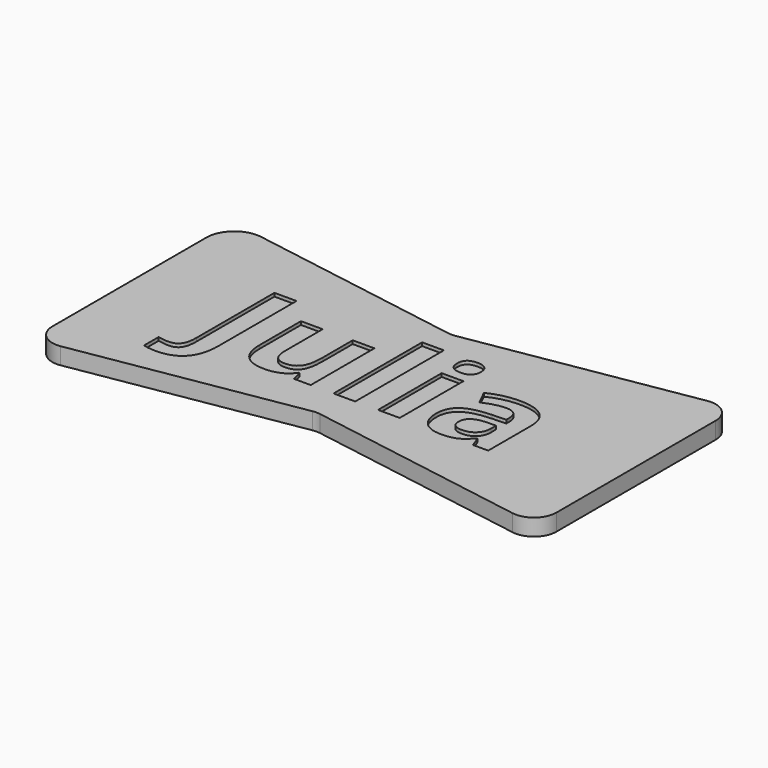
from build123d import *

# Parameters (mm, degrees)
F1_DEPTH     = 3
F2_TEXT_SIZE = 26.0301089535
F3_DEPTH     = 0.6


# Not quite as in the source:
# - Text() gives the source's letters only with a copy of the font that has no kerning and outlines rounded to 1/6400 em; it was checked with that copy


with BuildPart() as f1:
    # F0 (on Top) → F1 (new body)
    with BuildSketch(Plane.XY):
        with BuildLine():
            ThreePointArc((-40.8889098256, 19.2117940781), (-44.9427792428, 18.0949243713), (-46.7109047621, 14.2798244589))
            Line((-46.7109047621, 14.2798244589), (-46.7109047621, -20.0960317456))
            ThreePointArc((-46.7109047621, -20.0960317456), (-45.2964043467, -23.1481116755), (-42.0533088129, -24.041607441))
            Line((-42.0533088129, -24.041607441), (-2.3685007114, -17.4274727574))
            ThreePointArc((-2.3685007114, -17.4274727574), (-1.7109047621, -17.3730484527), (-1.0533088129, -17.4274727574))
            Line((-1.0533088129, -17.4274727574), (38.6314992886, -24.041607441))
            ThreePointArc((38.6314992886, -24.041607441), (41.8745948224, -23.1481116755), (43.2890952379, -20.0960317456))
            Line((43.2890952379, -20.0960317456), (43.2890952379, 15.4602848806))
            ThreePointArc((43.2890952379, 15.4602848806), (41.8745948224, 18.5123648105), (38.6314992886, 19.4058605759))
            Line((38.6314992886, 19.4058605759), (-1.0533088129, 12.7917258924))
            ThreePointArc((-1.0533088129, 12.7917258924), (-1.7109047621, 12.7373015877), (-2.3685007114, 12.7917258924))
            Line((-2.3685007114, 12.7917258924), (-40.8889098256, 19.2117940781))
        make_face()
    extrude(amount=F1_DEPTH)

    # F2 (on face) → F3 (cut)
    with BuildSketch(Plane.XY.offset(3)):
        with Locations((-31.2083055724, -11.4084417)):
            Text('Julia', F2_TEXT_SIZE, font='Open Sans', font_style=FontStyle.BOLD, text_align=(TextAlign.LEFT, TextAlign.BOTTOM))
    extrude(amount=-F3_DEPTH, mode=Mode.SUBTRACT)


solid = f1.part
